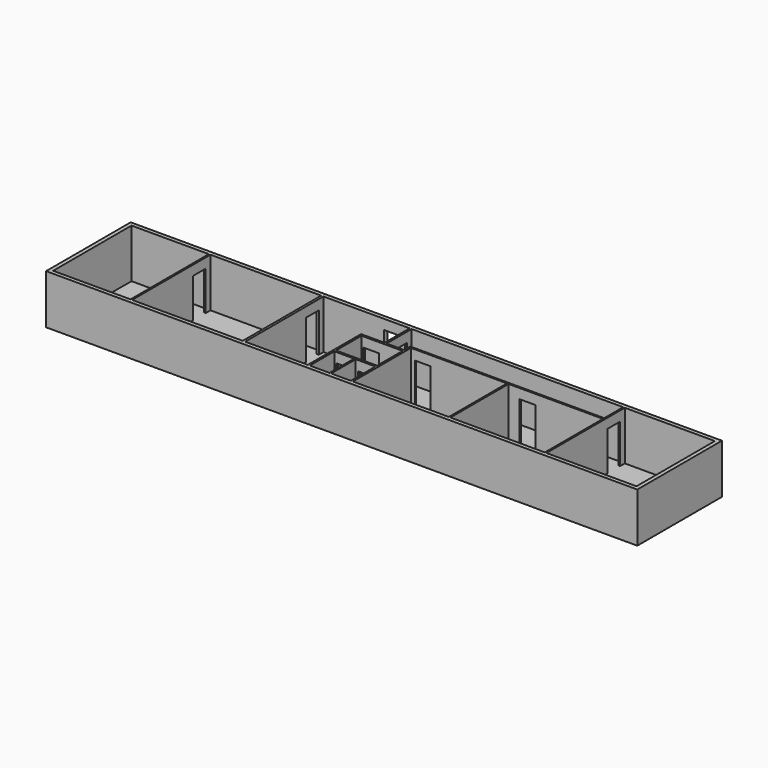
from build123d import *

# Parameters (mm, degrees)
F0_W          = 29780
F0_H          = 5000
F1_DEPTH      = 25
F2_W          = 30180
F2_H          = 5400
F2_W_2        = 29780
F2_H_2        = 5000
F3_DEPTH      = 2500
F3_DEPTH_BACK = 25
F4_W          = 80
F4_H          = 5000
F4_W_2        = 120
F4_W_3        = 100
F4_H_2        = 1600
F4_H_3        = 3710
F4_H_4        = 1570
F5_DEPTH      = 2500
F6_W          = 800
F6_H          = 2000
F7_DEPTH      = 21230
F8_W          = 800
F8_H          = 2000
F9_DEPTH      = 80
F10_W         = 800
F10_H         = 2000
F11_DEPTH     = 100
F12_W         = 800
F12_H         = 2000
F13_DEPTH     = 100
F14_TEXT_SIZE = 1527.0339945952
F15_DEPTH     = 25
F16_W         = 800
F16_H         = 2000
F17_DEPTH     = 225.0010001


# Not quite as in the source:
# - Text() gives the source's letters only with a copy of the font that has no kerning and outlines rounded to 1/6400 em; it was checked with that copy


with BuildPart() as f1:
    # F0 (on Top) → F1 (new body)
    with BuildSketch(Plane.XY):
        with Locations((-2077.1158394969, 1.5123458579)):
            Rectangle(F0_W, F0_H)
    extrude(amount=F1_DEPTH)

    # F2 (on face) → F3 (join, two sides)
    with BuildSketch(Plane.XY.offset(25)) as f3_sk:
        with Locations((-2077.1158394969, 1.5123458579)):
            Rectangle(F2_W, F2_H)
        with Locations((-2077.1158394969, 1.5123458579)):
            Rectangle(F2_W_2, F2_H_2, mode=Mode.SUBTRACT)
    extrude(amount=F3_DEPTH)
    extrude(f3_sk.sketch, amount=-F3_DEPTH_BACK)

    # F4 (on face) → F5 (join, through all)
    with BuildSketch(Plane.XY.offset(25)):
        with Locations((-12977.1158394969, 1.5123458579)):
            Rectangle(F4_W, F4_H)
        with Locations((-7227.1158394969, 1.5123458579)):
            Rectangle(F4_W_2, F4_H)
        with Locations((-2717.1158394969, 1701.5123458579)):
            Rectangle(F4_W_3, F4_H_2)
        Polygon((-2667.1158394969, 901.5123458579), (-2767.1158394969, 901.5123458579), (-3967.1158394969, 901.5123458579), (-3967.1158394969, 801.5123458579), (-3867.1158394969, 801.5123458579), (-1767.1158394969, 801.5123458579), (-1667.1158394969, 801.5123458579), (-1667.1158394969, 901.5123458579), (-1767.1158394969, 901.5123458579), align=None)
        Polygon((-1767.1158394969, 1291.5123458579), (-1767.1158394969, 901.5123458579), (-1667.1158394969, 901.5123458579), (-1667.1158394969, 1211.5123458579), (-1667.1158394969, 1291.5123458579), align=None)
        Polygon((-3867.1158394969, 801.5123458579), (-3967.1158394969, 801.5123458579), (-3967.1158394969, -2498.4876541421), (-3867.1158394969, -2498.4876541421), (-3867.1158394969, -928.4876541421), (-3867.1158394969, -828.4876541421), align=None)
        Polygon((-1667.1158394969, -2498.4876541421), (-1667.1158394969, 801.5123458579), (-1767.1158394969, 801.5123458579), (-1767.1158394969, -828.4876541421), (-1767.1158394969, -928.4876541421), (-1767.1158394969, -2498.4876541421), align=None)
        Polygon((-1667.1158394969, 1291.5123458579), (-1667.1158394969, 1211.5123458579), (3232.8841605031, 1211.5123458579), (3312.8841605031, 1211.5123458579), (8132.8841605031, 1211.5123458579), (8132.8841605031, 1291.5123458579), align=None)
        Polygon((-1767.1158394969, -828.4876541421), (-3867.1158394969, -828.4876541421), (-3867.1158394969, -928.4876541421), (-2857.1158394969, -928.4876541421), (-2777.1158394969, -928.4876541421), (-1767.1158394969, -928.4876541421), align=None)
        with Locations((3272.8841605031, -643.4876541421)):
            Rectangle(F4_W, F4_H_3)
        Polygon((8132.8841605031, 2501.5123458579), (8132.8841605031, 1291.5123458579), (8132.8841605031, 1211.5123458579), (8132.8841605031, -2498.4876541421), (8212.8841605031, -2498.4876541421), (8212.8841605031, 2501.5123458579), align=None)
        with Locations((-2817.1158394969, -1713.4876541421)):
            Rectangle(F4_W, F4_H_4)
    extrude(amount=F5_DEPTH)

    # F6 (on face) → F7 (cut, through all)
    with BuildSketch(Plane.YZ.offset(8212.8841605031)):
        with Locations((1801.5123458579, 1025)):
            Rectangle(F6_W, F6_H)
    extrude(amount=-F7_DEPTH, mode=Mode.SUBTRACT)

    # F8 (on face) → F9 (cut, through all)
    with BuildSketch(Plane(origin=(0, 1291.5123458579, 0), x_dir=(-1, 0, 0), z_dir=(0, 1, 0))):
        with Locations((1067.1158394969, 1025)):
            Rectangle(F8_W, F8_H)
        with Locations((-4276.3398647308, 1025)):
            Rectangle(F8_W, F8_H)
    extrude(amount=-F9_DEPTH, mode=Mode.SUBTRACT)

    # F10 (on face) → F11 (cut, through all)
    with BuildSketch(Plane(origin=(0, 901.5123458579, 0), x_dir=(-1, 0, 0), z_dir=(0, 1, 0))):
        with Locations((3367.1158394969, 1025)):
            Rectangle(F10_W, F10_H)
    extrude(amount=-F11_DEPTH, mode=Mode.SUBTRACT)

    # F12 (on face) → F13 (cut, through all)
    with BuildSketch(Plane(origin=(0, -828.4876541421, 0), x_dir=(-1, 0, 0), z_dir=(0, 1, 0))):
        with Locations((3367.1158394969, 1025)):
            Rectangle(F12_W, F12_H)
        with Locations((2267.1158394969, 1025)):
            Rectangle(F12_W, F12_H)
    extrude(amount=-F13_DEPTH, mode=Mode.SUBTRACT)

    # F14 (on face) → F15 (join)
    with BuildSketch(Plane(origin=(0, 2701.5123458579, 0), x_dir=(-1, 0, 0), z_dir=(0, 1, 0))):
        with Locations((-9814.2738342285, 822.9711651802)):
            Text('Bureaux Admin', F14_TEXT_SIZE, font='Open Sans', text_align=(TextAlign.LEFT, TextAlign.BOTTOM))
    extrude(amount=F15_DEPTH)

    # F16 (on face) → F17 (cut, through all)
    with BuildSketch(Plane.XZ.offset(-2501.5123458579)):
        with Locations((-3667.1158394969, 1025)):
            Rectangle(F16_W, F16_H)
    extrude(amount=-F17_DEPTH, mode=Mode.SUBTRACT)


solid = f1.part
